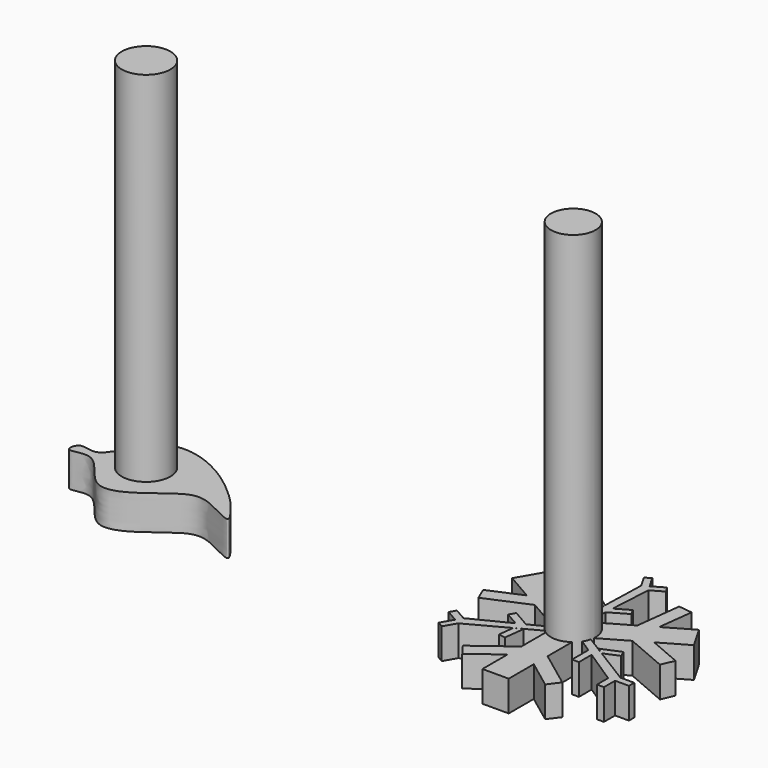
from build123d import *

# Parameters (mm, degrees)
F2_DEPTH  = 2
F1_R      = 1.4605
F3_DEPTH  = 25.4
F5_DEPTH  = 1
F7_SCALE  = 2.25
F9_R      = 1.5875
F10_DEPTH = 25.4


# Not quite as in the source:
# - ends of sketch curves that miss each other by under 0.0002 mm in the source are joined


with BuildPart() as f2:
    # F0 (on Top) → F2 (new body)
    with BuildSketch(Plane.XY):
        Polygon((-0.0127014339, 0.9898670365), (0.0557615141, 1.029394138), (0.138240911, 2.4622835197), (0.1693981397, 3.0035685424), (0.3253258613, 5.7124532465), (1.1109840408, 6.166053208), (0.8841841765, 6.5588820961), (0.0985259969, 6.1052821346), (-0.3550739645, 6.8909403142), (-0.7315351504, 6.6735903472), (-0.2779351889, 5.8879321677), (-0.3631976516, 3.0396497277), (-0.3593508306, 3.0367321709), (-0.3663883129, 2.9330623245), (-0.4175601747, 1.2236123396), align=None)
        Polygon((-0.8508992831, -0.9734238887), (-0.8508992831, -0.5059332827), (-0.9193622311, -0.4664061812), (-2.2015205349, -1.1114216191), (-2.6858657296, -1.3550811789), (-5.10979256, -2.5744861629), (-5.8954507396, -2.1208862014), (-6.1222506039, -2.5137150896), (-5.3365924243, -2.967315051), (-5.7901923858, -3.7529732306), (-5.4137312, -3.9703231976), (-4.9601312385, -3.184665018), (-2.450815057, -1.8343632567), (-2.4502117892, -1.8295730336), (-2.3569123275, -1.7838327489), align=None)
        Polygon((0, 1.348e-07), (0.0063507169, 1.348e-07), (0.8636007169, 1.348e-07), (1.2684594578, -0.2501884508), (3.1750801818, 0.8505995374), (4.151752869, 1.4144817763), (5.9247108388, 2.4380995374), (5.0674608388, 3.9229000922), (3.294502869, 2.8992823311), (2.3178301818, 2.3354000922), (0.0557615141, 1.029394138), (0.0513573913, 0.9528826566), (0.4254497583, 0.7369003278), align=None)
        Polygon((0.4254495248, -0.7369004626), (-1.167e-07, -6.74e-08), (-0.0031752417, -0.0054999496), (-0.4318002417, -0.747900227), (-0.8508992831, -0.9734238887), (-0.8508992831, -3.1749998652), (-0.8508992831, -4.3027643429), (-0.8508992831, -6.3499998652), (0.8636007169, -6.3499998652), (0.8636007169, -4.3027643429), (0.8636007169, -3.1749998652), (0.8636007169, -0.5629879568), (0.7995418918, -0.5209181338), align=None)
        Polygon((-0.8508992831, -4.3027643429), (-0.8508992831, -3.1749998652), (-3.2412230885, -4.9631580294), (-2.7002857532, -5.6862570345), align=None)
        Polygon((3.2539245223, -4.9631580294), (0.8636007169, -3.1749998652), (0.8636007169, -4.3027643429), (2.7129871871, -5.6862570345), align=None)
        Polygon((2.5164675899, -1.6484873635), (2.0632796239, -1.3508619006), (2.0632796239, -2.6843671221), (2.5164675899, -2.6843671221), align=None)
        Polygon((2.359458579, -0.90489005), (2.7233006404, -1.1492295757), (2.8140127086, -1.205286471), (3.7643470012, -0.8053710598), (3.5885683743, -0.3876615832), align=None)
        Polygon((0.1693981397, 3.0035685424), (0.138240911, 2.4622835197), (1.2930903089, 3.1290361305), (1.0664963259, 3.5215084217), align=None)
        Polygon((-0.3960715185, 2.4957960936), (-0.3663883129, 2.9330623245), (-0.3631976516, 3.0396497277), (-1.1847017034, 3.6627056616), (-1.458559408, 3.301622167), align=None)
        Polygon((4.151752869, 1.4144817763), (3.1750801818, 0.8505995374), (5.9188324807, -0.3254025192), (6.274585921, 0.5046124575), align=None)
        Polygon((2.6712586753, 5.299560313), (2.3178301818, 2.3354000922), (3.294502869, 2.8992823311), (3.5679494508, 5.1926443415), align=None)
        Polygon((-2.6858657296, -1.3550811789), (-2.2015205349, -1.1114216191), (-3.3563699328, -0.4446690084), (-3.5829639158, -0.8371412996), align=None)
        Polygon((-1.9633870605, -1.5909060436), (-2.3569123275, -1.7838327489), (-2.450815057, -1.8343632567), (-2.5796452979, -2.8573346018), (-2.1300089663, -2.9139605838), align=None)
        Polygon((-3.3008535859, 2.8882825667), (-2.3241808987, 2.3244003278), (-2.6776093922, 5.2885605486), (-3.5743001677, 5.181644577), align=None)
        Polygon((-5.9251831976, -0.3364022836), (-3.1814308987, 0.839599773), (-4.1581035859, 1.4034820119), (-6.2809366379, 0.4936126931), align=None)
        Polygon((0.8636007169, 1.348e-07), (0.0063507169, 1.348e-07), (0.7995418918, -0.5209181338), (0.8636007169, -0.4839337539), align=None)
        Polygon((-0.8508992831, 1.348e-07), (0, 1.348e-07), (-0.0031754752, 0.0054998148), (-0.4318004752, 0.7479000922), (-0.4175601747, 1.2236123396), (-2.3241808987, 2.3244003278), (-3.3008535859, 2.8882825667), (-5.0738115558, 3.9119003278), (-5.9310615558, 2.427099773), (-4.1581035859, 1.4034820119), (-3.1814308987, 0.839599773), (-0.9193622311, -0.4664061812), (-0.8508992831, -0.4319645227), align=None)
        Polygon((1.2684594578, -0.2501884508), (0.8636007169, -0.4839337539), (0.8636007169, -0.5629879568), (2.0632796239, -1.3508619006), (2.5164675899, -1.6484873635), (4.7844666988, -3.1379670836), (4.7844666988, -4.0451670066), (5.2380664274, -4.0451670066), (5.2380664274, -3.1379670836), (6.1452663504, -3.1379670836), (6.1452663504, -2.7032671496), (5.2380664274, -2.7032671496), (2.8140127086, -1.205286471), (2.8095626198, -1.2071591373), (2.7233006404, -1.1492295757), align=None)
        Polygon((0.7995418918, -0.5209181338), (0.0063507169, 1.348e-07), (0, 1.348e-07), (0.4254495248, -0.7369004626), align=None)
        Polygon((-0.4318004752, 0.7479000922), (-0.0031754752, 0.0054998148), (0.0513573913, 0.9528826566), (-0.0127014339, 0.9898670365), align=None)
        Polygon((-0.0031754752, 0.0054998148), (-1.167e-07, -6.74e-08), (0.4254497583, 0.7369003278), (0.0513573913, 0.9528826566), align=None)
        Polygon((-0.4318002417, -0.747900227), (-0.0031752417, -0.0054999496), (-0.8508992831, -0.4319645227), (-0.8508992831, -0.5059332827), align=None)
        Polygon((-0.0031752417, -0.0054999496), (1.167e-07, -6.74e-08), (-0.8508992831, 1.348e-07), (-0.8508992831, -0.4319645227), align=None)
        Polygon((1.2684594578, -0.2501884508), (0.8636007169, 1.348e-07), (0.8636007169, -0.4839337539), align=None)
        Polygon((-0.8508992831, -0.9734238887), (-0.4318002417, -0.747900227), (-0.8508992831, -0.5059332827), align=None)
        Polygon((-0.0127014339, 0.9898670365), (0.0513573913, 0.9528826566), (0.0557615141, 1.029394138), align=None)
        Polygon((-0.8508992831, -0.5059332827), (-0.8508992831, -0.4319645227), (-0.9193622311, -0.4664061812), align=None)
        Polygon((-0.3631976516, 3.0396497277), (-0.3663883129, 2.9330623245), (-0.3593508306, 3.0367321709), align=None)
        Polygon((2.8140127086, -1.205286471), (2.7233006404, -1.1492295757), (2.8095626198, -1.2071591373), align=None)
        Polygon((-0.4175601747, 1.2236123396), (-0.4318004752, 0.7479000922), (-0.0127014339, 0.9898670365), align=None)
        Polygon((0.8636007169, -0.4839337539), (0.7995418918, -0.5209181338), (0.8636007169, -0.5629879568), align=None)
        Polygon((-2.450815057, -1.8343632567), (-2.3569123275, -1.7838327489), (-2.4502117892, -1.8295730336), align=None)
    extrude(amount=F2_DEPTH)

    # F1 (on Top) → F3 (join)
    with BuildSketch(Plane.XY):
        Circle(F1_R)
    extrude(amount=F3_DEPTH)


with BuildPart() as f5:
    # F4 (on Top) → F5 (new body)
    with BuildSketch(Plane.XY):
        with BuildLine():
            add(Edge.make_bspline(
                [(-29.8669375479, 0.2857499931), (-29.7440304745, 0.3571436979), (-29.1547614666, -0.031081706), (-28.6573535606, 1.9086215428), (-26.8097076406, 1.4876465764), (-25.6137182394, 0.4424417951), (-25.3000873709, 0.0757578444), (-24.7765698555, -0.6160305024), (-25.5747691832, -0.1631625611), (-26.2801418295, 0.1338939544), (-26.9852315195, -0.4157522042), (-28.4156101147, -1.4829106615), (-29.1578723902, 0.3232844338), (-30.049192476, -0.1925589818), (-29.9590967439, 0.2322169762), (-29.8669375479, 0.2857499931)],
                knots=[0, 0, 0, 0, 0.0595602967, 0.1590621278, 0.2623182491, 0.3653254409, 0.4276419031, 0.4859643703, 0.5478739218, 0.6200200353, 0.696962825, 0.7939279281, 0.8918484857, 0.9553400069, 1, 1, 1, 1], degree=3))
        make_face()
    extrude(amount=F5_DEPTH)


with BuildPart() as f5_1:
    # F7: moved
    add(f5.part.scale(F7_SCALE).moved(Location((34.892889671, -0.5655468703, -1.25))))


with BuildPart() as f5_2:
    # F8: moved
    add(f5_1.part.moved(Location((0, 0, 1))))

    # F9 (on Top) → F10 (join)
    with BuildSketch(Plane.XY):
        with Locations((-28.1345900148, 0.302218803)):
            Circle(F9_R)
    extrude(amount=F10_DEPTH)


solid = Compound([f2.part, f5_2.part])
